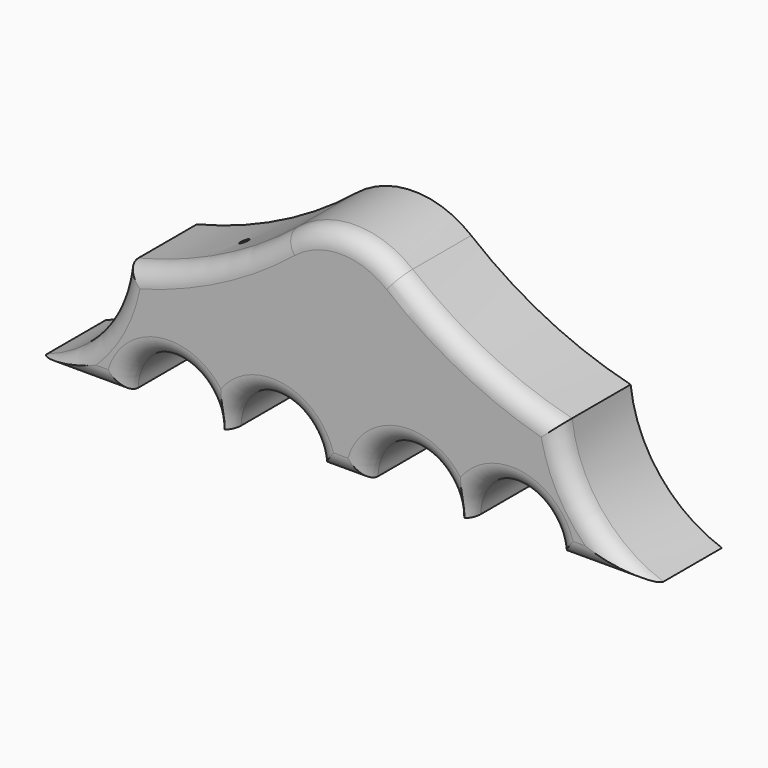
from build123d import *

# Parameters (mm, degrees)
F1_DEPTH      = 25.4
F2_T          = -2.54
F3_R          = 1.25
F4_DEPTH      = 2.54
F8_R          = 1.25
F9_REACH      = 97.0761529787
F10_T3_ANGLE  = 102.7022432279
F10_T6_ANGLE  = 31.3976037726
F10_T9_ANGLE  = 102.7022432279
F10_T12_ANGLE = 294.7758439205
F10_T15_ANGLE = 294.7758439205
F10_T18_ANGLE = 294.7758439205
F10_T21_ANGLE = 294.7758439205
F10_T24_DEPTH = 50.8
F10_T27_DEPTH = 38.1
F10_T30_DEPTH = 50.8
F10_T33_ANGLE = 31.3976037726
F10_T36_ANGLE = 77.9901739098


# Not quite as in the source:
# - a fillet or chamfer that OpenCascade refuses, or shapes differently, is made with other operations: its cross-section is extruded or revolved along the edge and cut away or added


with BuildPart() as f1:
    # F0 (on Front) → F1 (new body)
    with BuildSketch(Plane.XZ):
        with BuildLine():
            ThreePointArc((-50.0310228288, -3.8065822828), (-58.1416465627, -23.3530832956), (-75.4310228288, -35.5565822828))
            Line((-75.4310228288, -35.5565822828), (-50.0310228288, -35.5565822828))
            ThreePointArc((-50.0310228288, -35.5565822828), (-37.3310228288, -22.8565822828), (-24.6310228288, -35.5565822828))
            Line((-24.6310228288, -35.5565822828), (-21.4560228288, -35.5565822828))
            ThreePointArc((-21.4560228288, -35.5565822828), (-8.7560228288, -22.8565822828), (3.9439771712, -35.5565822828))
            Line((3.9439771712, -35.5565822828), (16.6439771712, -35.5565822828))
            ThreePointArc((16.6439771712, -35.5565822828), (29.3439771712, -22.8565822828), (42.0439771712, -35.5565822828))
            Line((42.0439771712, -35.5565822828), (45.2189771712, -35.5565822828))
            ThreePointArc((45.2189771712, -35.5565822828), (57.9189771712, -22.8565822828), (70.6189771712, -35.5565822828))
            Line((70.6189771712, -35.5565822828), (96.0189771712, -35.5565822828))
            ThreePointArc((96.0189771712, -35.5565822828), (78.7296009051, -23.3530832956), (70.6189771712, -3.8065822828))
            ThreePointArc((70.6189771712, -3.8065822828), (47.2369488247, 4.8063759681), (26.2770224058, 18.2816787082))
            ThreePointArc((26.2770224058, 18.2816787082), (10.2939771712, 23.9408006875), (-5.6890680634, 18.2816787082))
            ThreePointArc((-5.6890680634, 18.2816787082), (-26.6489944823, 4.8063759681), (-50.0310228288, -3.8065822828))
        make_face()
    extrude(amount=F1_DEPTH)

    # F2
    f2_openings = [f1.faces().sort_by_distance(p)[0] for p in [
        (10.293977, 0, -9.758382),
    ]]
    offset(amount=F2_T, openings=f2_openings)

    # F3 (on face) → F4 (cut, through all)
    with BuildSketch(Plane(origin=(0, 0, -35.5565822828), x_dir=(1, 0, 0), z_dir=(0, 0, -1))):
        with Locations((10.2939771712, 12.7)):
            Circle(F3_R)
    extrude(amount=-F4_DEPTH, mode=Mode.SUBTRACT)

    f9_end = f1.faces().sort_by_distance((-24.7436453576, -11.43, 2.9213828953))[0]
    # F8 (on line) → F9 (cut, up to a face of the model that its end follows)
    with BuildSketch(Plane(origin=(-8.427281394, 0, 16.9176799622), x_dir=(0.8950940843, 0, 0.4458773153), z_dir=(-0.4458773153, 0, 0.8950940843))):
        with Locations((-21.7103033003, -12.7)):
            Circle(F8_R)
    f9_long = extrude(amount=-F9_REACH, mode=Mode.PRIVATE)
    add(split(f9_long, bisect_by=f9_end, keep=Keep.BOTTOM, mode=Mode.PRIVATE), mode=Mode.SUBTRACT)

    # F10: fillet of radius 5.08 on 14 edges, made by hand


with BuildPart() as f10_tool1:
    # F10_s2 → F10_t3 (revolve)
    with BuildSketch(Plane(origin=(108.4807840202, 0, 0.0206940316), x_dir=(0, 1, 0), z_dir=(0.9999999818, 0, 0.0001907622))):
        with BuildLine():
            ThreePointArc((-25.4, -42.7528960076), (-23.9121024484, -39.1607935592), (-20.32, -37.6728960076))
            Line((-20.32, -37.6728960076), (-25.4, -37.6728960076))
            Line((-25.4, -37.6728960076), (-25.4, -42.7528960076))
        make_face()
    revolve(axis=Axis((108.4807025449, -25.4, 0.4477980162), (0, 1, 0)), revolution_arc=F10_T3_ANGLE)


with BuildPart() as f10_tool4:
    # F10_s5 → F10_t6 (revolve)
    with BuildSketch(Plane(origin=(82.44641514, 0, -10.9970144086), x_dir=(0, 1, 0), z_dir=(0.9912213489, 0, -0.1322128492))):
        with BuildLine():
            ThreePointArc((-25.4, -0.2213031635), (-23.9121024484, 3.370799285), (-20.32, 4.8586968365))
            Line((-20.32, 4.8586968365), (-25.4, 4.8586968365))
            Line((-25.4, 4.8586968365), (-25.4, -0.2213031635))
        make_face()
    revolve(axis=Axis((98.2007259613, -25.4, 107.1156298016), (0, 1, 0)), revolution_arc=F10_T6_ANGLE)


with BuildPart() as f10_tool7:
    # F10_s8 → F10_t9 (revolve)
    with BuildSketch(Plane(origin=(-4.3383262672, 0, 19.2642896077), x_dir=(0, 1, 0), z_dir=(-0.2196983006, 0, 0.9755678637))):
        with BuildLine():
            ThreePointArc((-20.32, 47.5469601373), (-23.9121024484, 46.0590625857), (-25.4, 42.4669601373))
            Line((-25.4, 42.4669601373), (-25.4, 47.5469601373))
            Line((-25.4, 47.5469601373), (-20.32, 47.5469601373))
        make_face()
    revolve(axis=Axis((-87.8927482025, -25.4, 0.4477980162), (0, 1, 0)), revolution_arc=F10_T9_ANGLE)


with BuildPart() as f10_tool10:
    # F10_s11 → F10_t12 (revolve)
    with BuildSketch(Plane(origin=(57.2373966966, 0, -36.6218451563), x_dir=(0, 1, 0), z_dir=(0.8423388046, 0, -0.5389483633))):
        with BuildLine():
            ThreePointArc((-25.4, -16.5153510633), (-23.9121024484, -12.9232486148), (-20.32, -11.4353510633))
            Line((-20.32, -11.4353510633), (-25.4, -11.4353510633))
            Line((-25.4, -11.4353510633), (-25.4, -16.5153510633))
        make_face()
    revolve(axis=Axis((57.9189771712, -25.4, -35.5565822828), (0, 1, 0)), revolution_arc=F10_T12_ANGLE)


with BuildPart() as f10_tool13:
    # F10_s14 → F10_t15 (revolve)
    with BuildSketch(Plane(origin=(36.9624437391, 0, -23.6494489501), x_dir=(0, 1, 0), z_dir=(0.8423388046, 0, -0.5389483633))):
        with BuildLine():
            ThreePointArc((-25.4, -31.915800545), (-23.9121024484, -28.3236980966), (-20.32, -26.835800545))
            Line((-20.32, -26.835800545), (-25.4, -26.835800545))
            Line((-25.4, -26.835800545), (-25.4, -31.915800545))
        make_face()
    revolve(axis=Axis((29.3439771712, -25.4, -35.5565822828), (0, 1, 0)), revolution_arc=F10_T15_ANGLE)


with BuildPart() as f10_tool16:
    # F10_s17 → F10_t18 (revolve)
    with BuildSketch(Plane(origin=(9.929173129, 0, -6.3529206751), x_dir=(0, 1, 0), z_dir=(0.8423388046, 0, -0.5389483633))):
        with BuildLine():
            ThreePointArc((-25.4, -52.4497331873), (-23.9121024484, -48.8576307389), (-20.32, -47.3697331873))
            Line((-20.32, -47.3697331873), (-25.4, -47.3697331873))
            Line((-25.4, -47.3697331873), (-25.4, -52.4497331873))
        make_face()
    revolve(axis=Axis((-8.7560228288, -25.4, -35.5565822828), (0, 1, 0)), revolution_arc=F10_T18_ANGLE)


with BuildPart() as f10_tool19:
    # F10_s20 → F10_t21 (revolve)
    with BuildSketch(Plane(origin=(-10.3457798285, 0, 6.6194755311), x_dir=(0, 1, 0), z_dir=(0.8423388046, 0, -0.5389483633))):
        with BuildLine():
            ThreePointArc((-25.4, -67.850182669), (-23.9121024484, -64.2580802206), (-20.32, -62.770182669))
            Line((-20.32, -62.770182669), (-25.4, -62.770182669))
            Line((-25.4, -62.770182669), (-25.4, -67.850182669))
        make_face()
    revolve(axis=Axis((-37.3310228288, -25.4, -35.5565822828), (0, 1, 0)), revolution_arc=F10_T21_ANGLE)


with BuildPart() as f10_tool22:
    # F10_s23 → F10_t24 (new body)
    with BuildSketch(Plane.YZ.offset(57.9189771712)):
        with BuildLine():
            ThreePointArc((-25.4, -30.4765822828), (-23.9121024484, -34.0686847312), (-20.32, -35.5565822828))
            Line((-20.32, -35.5565822828), (-25.4, -35.5565822828))
            Line((-25.4, -35.5565822828), (-25.4, -30.4765822828))
        make_face()
    extrude(amount=F10_T24_DEPTH)


with BuildPart() as f10_tool25:
    # F10_s26 → F10_t27 (new body)
    with BuildSketch(Plane.YZ.offset(-8.7560228288)):
        with BuildLine():
            ThreePointArc((-25.4, -30.4765822828), (-23.9121024484, -34.0686847312), (-20.32, -35.5565822828))
            Line((-20.32, -35.5565822828), (-25.4, -35.5565822828))
            Line((-25.4, -35.5565822828), (-25.4, -30.4765822828))
        make_face()
    extrude(amount=F10_T27_DEPTH)


with BuildPart() as f10_tool28:
    # F10_s29 → F10_t30 (new body)
    with BuildSketch(Plane.YZ.offset(-88.1310228288)):
        with BuildLine():
            ThreePointArc((-20.32, -35.5565822828), (-23.9121024484, -34.0686847312), (-25.4, -30.4765822828))
            Line((-25.4, -30.4765822828), (-25.4, -35.5565822828))
            Line((-25.4, -35.5565822828), (-20.32, -35.5565822828))
        make_face()
    extrude(amount=F10_T30_DEPTH)


with BuildPart() as f10_tool31:
    # F10_s32 → F10_t33 (revolve)
    with BuildSketch(Plane(origin=(5.5043409487, 0, 4.4565459691), x_dir=(0, 1, 0), z_dir=(0.7771999221, 0, 0.6292537494))):
        with BuildLine():
            ThreePointArc((-20.32, 17.7883866769), (-23.9121024484, 16.3004891253), (-25.4, 12.7083866769))
            Line((-25.4, 12.7083866769), (-25.4, 17.7883866769))
            Line((-25.4, 17.7883866769), (-20.32, 17.7883866769))
        make_face()
    revolve(axis=Axis((-77.612771619, -25.4, 107.1156298016), (0, 1, 0)), revolution_arc=F10_T33_ANGLE)


with BuildPart() as f10_tool34:
    # F10_s35 → F10_t36 (revolve)
    with BuildSketch(Plane(origin=(6.9316012045, 0, -5.6121159091), x_dir=(0, 1, 0), z_dir=(0.7771999221, 0, -0.6292537494))):
        with BuildLine():
            ThreePointArc((-25.4, 25.6634341392), (-23.9121024484, 29.2555365876), (-20.32, 30.7434341392))
            Line((-20.32, 30.7434341392), (-25.4, 30.7434341392))
            Line((-25.4, 30.7434341392), (-25.4, 25.6634341392))
        make_face()
    revolve(axis=Axis((10.2939771712, -25.4, -1.4591993125), (0, -1, 0)), revolution_arc=F10_T36_ANGLE)


with BuildPart() as f1_1:
    add(f1.part)

    # F10_t37: cut F10_tool1, F10_tool4, F10_tool7, F10_tool10, F10_tool13, F10_tool16, F10_tool19, F10_tool22, F10_tool25, F10_tool28, F10_tool31, F10_tool34
    add([f10_tool1.part, f10_tool4.part, f10_tool7.part, f10_tool10.part, f10_tool13.part, f10_tool16.part, f10_tool19.part, f10_tool22.part, f10_tool25.part, f10_tool28.part, f10_tool31.part, f10_tool34.part], mode=Mode.SUBTRACT)


solid = f1_1.part
